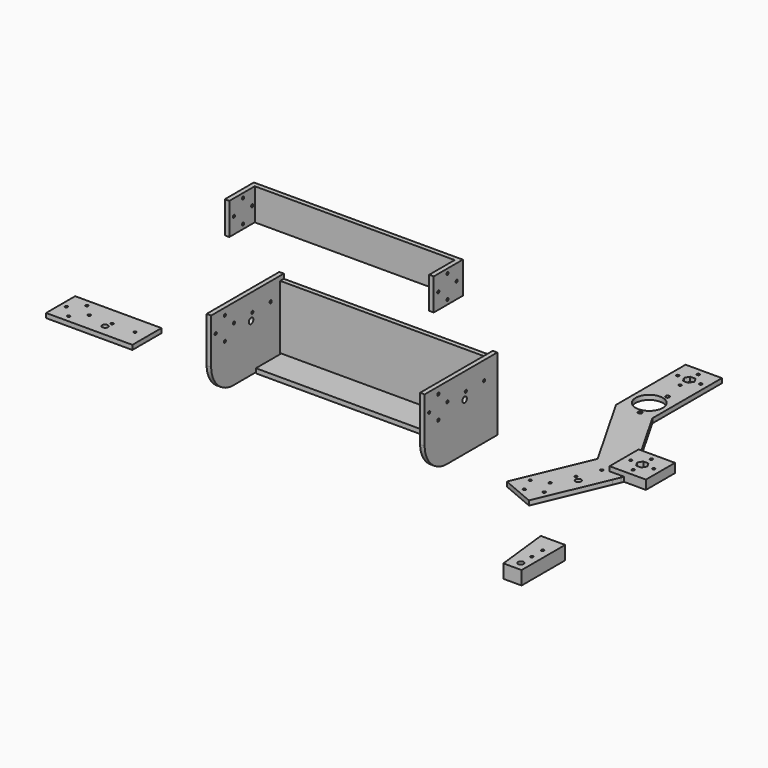
from build123d import *

# Parameters (mm, degrees)
F0_R      = 19.05
F0_R_2    = 2.703776852
F0_R_3    = 1.905
F1_DEPTH  = 6.35
F2_W      = 50.8
F2_H      = 50.8
F2_R      = 1.905
F3_DEPTH  = 12.7
F4_R      = 3.96875
F4_R_2    = 1.905
F5_DEPTH  = 19.05
F7_DEPTH  = 6.35
F8_W      = 6.35
F8_H      = 101.6
F9_DEPTH  = 120.65
F10_W     = 144.4625
F10_H     = 6.35
F11_DEPTH = 44.45
F14_DEPTH = 44.45
F12_R     = 3.96875
F12_R_2   = 1.905
F15_DEPTH = 527.1911687145
F17_R     = 1.905
F18_DEPTH = 292.101
F16_R     = 3.96875
F16_R_2   = 1.905
F19_DEPTH = 6.35
F20_W     = 120.65
F20_H     = 50.8
F20_R     = 1.905
F20_R_2   = 3.96875
F21_DEPTH = 6.35
F22_W     = 292.1
F22_H     = 6.35
F23_DEPTH = 6.35


# Not quite as in the source:
# - a feature names something its author has since deleted; it is built from what else it names


with BuildPart() as f1:
    # F0 (on Top) → F1 (new body)
    with BuildSketch(Plane.XY):
        Polygon((-41.9181553716, 248.7370216466), (-92.7181553716, 248.7370216466), (-92.7181553716, 127.1085888147), (-28.5808505793, 14.8683054282), (-42.2464598706, -17.3884454803), (-48.4258579806, -31.9744987877), (-72.5243088059, -88.8572699093), (-25.7488163324, -108.6737606142), (14.6531866834, -13.3075519289), (18.7877209912, -3.5482619883), (24.7290826448, 10.4759222859), (-41.9181553716, 127.1085888147), align=None)
        with Locations((-67.3181553716, 153.4870216466)):
            Circle(F0_R, mode=Mode.SUBTRACT)
        with Locations((-60.8181553716, 129.4870216466)):
            Circle(F0_R_2, mode=Mode.SUBTRACT)
        with Locations((-83.3181553716, 223.3370216466)):
            Circle(F0_R_3, mode=Mode.SUBTRACT)
        with Locations((-67.3181553716, 207.3370216466)):
            Circle(F0_R_3, mode=Mode.SUBTRACT)
        Polygon((-74.6505037903, 223.3370216466), (-70.984329581, 229.6870216466), (-63.6519811623, 229.6870216466), (-59.9858069529, 223.3370216466), (-63.6519811623, 216.9870216466), (-70.984329581, 216.9870216466), align=None, mode=Mode.SUBTRACT)
        with Locations((-67.3181553716, 239.3370216466)):
            Circle(F0_R_3, mode=Mode.SUBTRACT)
        with Locations((-60.8181553716, 177.4870216466)):
            Circle(F0_R_2, mode=Mode.SUBTRACT)
        with Locations((-51.3181553716, 223.3370216466)):
            Circle(F0_R_3, mode=Mode.SUBTRACT)
    extrude(amount=F1_DEPTH)

    # F16 (on face) → F19 (cut, through all)
    with BuildSketch(Plane.XY.offset(6.35)):
        with Locations((-13.1184830111, -38.1648051178)):
            Circle(F16_R)
        with Locations((-46.0158553715, -91.3992959746)):
            Circle(F16_R_2)
        with Locations((-33.533026581, -61.9344188259)):
            Circle(F16_R_2)
        with Locations((-54.5068795506, -70.425443005)):
            Circle(F16_R_2)
        with Locations((-25.0420024019, -82.9082717955)):
            Circle(F16_R_2)
        with Locations((-21.0501977905, -32.4695416772)):
            Circle(F16_R_2)
        with Locations((-8.567369, -3.0046645286)):
            Circle(F16_R_2)
    extrude(amount=-F19_DEPTH, mode=Mode.SUBTRACT)


with BuildPart() as f3:
    # F2 (on Top) → F3 (new body)
    with BuildSketch(Plane.XY):
        with Locations((25.4, 25.4)):
            Rectangle(F2_W, F2_H)
        with Locations((25.4, 9.4)):
            Circle(F2_R, mode=Mode.SUBTRACT)
        with Locations((9.4, 25.4)):
            Circle(F2_R, mode=Mode.SUBTRACT)
        Polygon((18.0676515813, 25.4), (21.7338257906, 31.75), (29.0661742094, 31.75), (32.7323484187, 25.4), (29.0661742094, 19.05), (21.7338257906, 19.05), align=None, mode=Mode.SUBTRACT)
        with Locations((41.4, 25.4)):
            Circle(F2_R, mode=Mode.SUBTRACT)
        with Locations((25.4, 41.4)):
            Circle(F2_R, mode=Mode.SUBTRACT)
    extrude(amount=F3_DEPTH)


with BuildPart() as f5:
    # F4 (on Top) → F5 (new body)
    with BuildSketch(Plane.XY):
        Polygon((51.9637279212, -185.1316541433), (60.6456212738, -261.3316541433), (86.0456212738, -261.3316541433), (86.0456212738, -185.1316541433), align=None)
        with Locations((74.9331212738, -248.6316541433)):
            Circle(F4_R, mode=Mode.SUBTRACT)
        with Locations((74.9331212738, -229.5816541433)):
            Circle(F4_R_2, mode=Mode.SUBTRACT)
        with Locations((74.9331212738, -210.5316541433)):
            Circle(F4_R_2, mode=Mode.SUBTRACT)
    extrude(amount=F5_DEPTH)


with BuildPart() as f7:
    # F6 (on Front) → F7 (new body)
    with BuildSketch(Plane.XZ):
        Polygon((-163.2913282394, 0), (-156.9413282394, 0), (-156.9413282394, 101.6), (-163.2913282394, 101.6), (-455.3913282394, 101.6), (-461.7413282394, 101.6), (-461.7413282394, 0), (-455.3913282394, 0), align=None)
    extrude(amount=F7_DEPTH)

    # F8 (on face) → F9 (join)
    with BuildSketch(Plane.XZ.offset(6.35)):
        with Locations((-458.5663282394, 50.8)):
            Rectangle(F8_W, F8_H)
        with Locations((-160.1163282394, 50.8)):
            Rectangle(F8_W, F8_H)
    extrude(amount=F9_DEPTH)

    # F10 (on face) → F11 (join)
    with BuildSketch(Plane.XZ.offset(6.35)):
        with Locations((-381.5725782394, 3.175)):
            Rectangle(F10_W, F10_H)
        with Locations((-237.1100782394, 3.175)):
            Rectangle(F10_W, F10_H)
    extrude(amount=F11_DEPTH)

    # F12 (on face) → F15 (cut, through all)
    with BuildSketch(Plane.YZ.offset(-156.9413282394)):
        with Locations((-57.15, 66.675)):
            Circle(F12_R)
        with Locations((-119, 76.2)):
            Circle(F12_R_2)
        with Locations((-103, 92.2)):
            Circle(F12_R_2)
        with Locations((-103, 60.2)):
            Circle(F12_R_2)
        with Locations((-87, 76.2)):
            Circle(F12_R_2)
        with Locations((-55, 76.2)):
            Circle(F12_R_2)
        with Locations((-23, 76.2)):
            Circle(F12_R_2)
        with BuildLine():
            ThreePointArc((-88.9, 0), (-115.5886324972, 11.4113675028), (-127, 38.1))
            Line((-127, 38.1), (-127, 0))
            Line((-127, 0), (-88.9, 0))
        make_face()
    extrude(amount=-F15_DEPTH, mode=Mode.SUBTRACT)

    # F22 (on face) → F23 (cut, through all)
    with BuildSketch(Plane(origin=(0, 0, 0), x_dir=(-1, 0, 0), z_dir=(0, 1, 0))):
        with Locations((309.3413282394, 98.425)):
            Rectangle(F22_W, F22_H)
    extrude(amount=-F23_DEPTH, mode=Mode.SUBTRACT)


with BuildPart() as f14:
    # F13 (on Top) → F14 (new body)
    with BuildSketch(Plane.XY):
        Polygon((-392.031496954, 233.5764824714), (-684.131496954, 233.5764824714), (-684.131496954, 182.7764824714), (-677.781496954, 182.7764824714), (-677.781496954, 227.2264824714), (-398.381496954, 227.2264824714), (-398.381496954, 182.7764824714), (-392.031496954, 182.7764824714), align=None)
    extrude(amount=F14_DEPTH)

    # F17 (on face) → F18 (cut, through all)
    with BuildSketch(Plane.YZ.offset(-392.031496954)):
        with Locations((206.7764824714, 38.225)):
            Circle(F17_R)
        with Locations((206.7764824714, 6.225)):
            Circle(F17_R)
        with Locations((222.7764824714, 22.225)):
            Circle(F17_R)
        with Locations((190.7764824714, 22.225)):
            Circle(F17_R)
    extrude(amount=-F18_DEPTH, mode=Mode.SUBTRACT)


with BuildPart() as f21:
    # F20 (on Top) → F21 (new body)
    with BuildSketch(Plane.XY):
        with Locations((-653.9018452168, -66.4971898071)):
            Rectangle(F20_W, F20_H)
        with Locations((-690.2268452168, -82.4971898071)):
            Circle(F20_R, mode=Mode.SUBTRACT)
        with Locations((-706.2268452168, -66.4971898071)):
            Circle(F20_R, mode=Mode.SUBTRACT)
        with Locations((-674.2268452168, -66.4971898071)):
            Circle(F20_R, mode=Mode.SUBTRACT)
        with Locations((-644.3768452168, -76.0221898071)):
            Circle(F20_R_2, mode=Mode.SUBTRACT)
        with Locations((-642.2268452168, -66.4971898071)):
            Circle(F20_R, mode=Mode.SUBTRACT)
        with Locations((-610.2268452168, -66.4971898071)):
            Circle(F20_R, mode=Mode.SUBTRACT)
        with Locations((-690.2268452168, -50.4971898071)):
            Circle(F20_R, mode=Mode.SUBTRACT)
    extrude(amount=F21_DEPTH)


solid = Compound([f1.part, f3.part, f5.part, f7.part, f14.part, f21.part])
